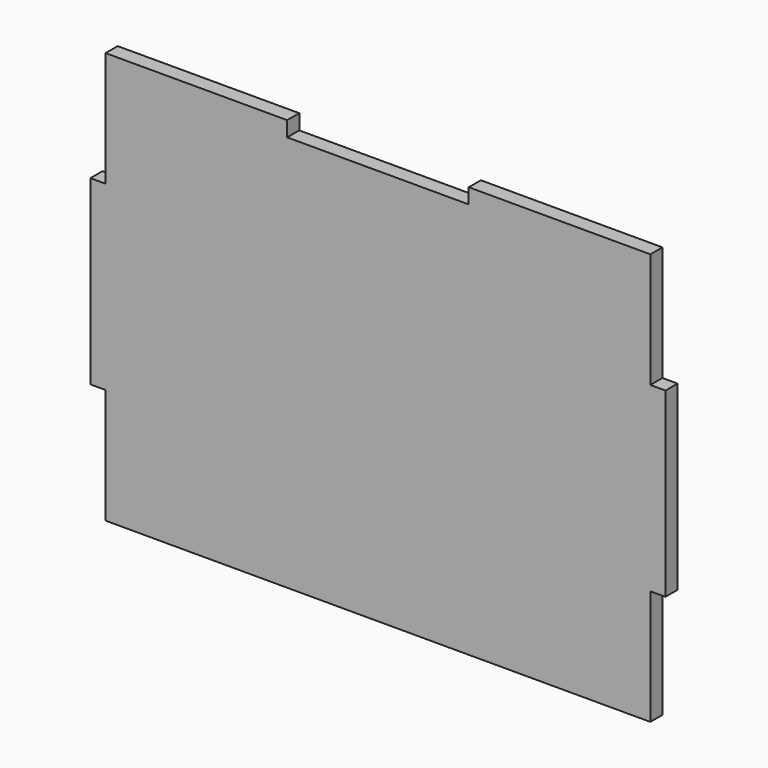
from build123d import *

# Parameters (mm, degrees)
F1_DEPTH = 3.175


# Not quite as in the source:
# - a feature names something its author has since deleted; it is built from what else it names


with BuildPart() as f1:
    # F0 (on Front) → F1 (new body)
    with BuildSketch(Plane.XZ):
        Polygon((-57.15, -43.18), (57.15, -43.18), (57.15, -19.05), (60.325, -19.05), (60.325, 19.05), (57.15, 19.05), (57.15, 43.18), (19.05, 43.18), (19.05, 40.005), (-19.05, 40.005), (-19.05, 43.18), (-57.15, 43.18), (-57.15, 19.05), (-60.325, 19.05), (-60.325, 0), (-60.325, -19.05), (-57.15, -19.05), align=None)
    extrude(amount=F1_DEPTH)


solid = f1.part
